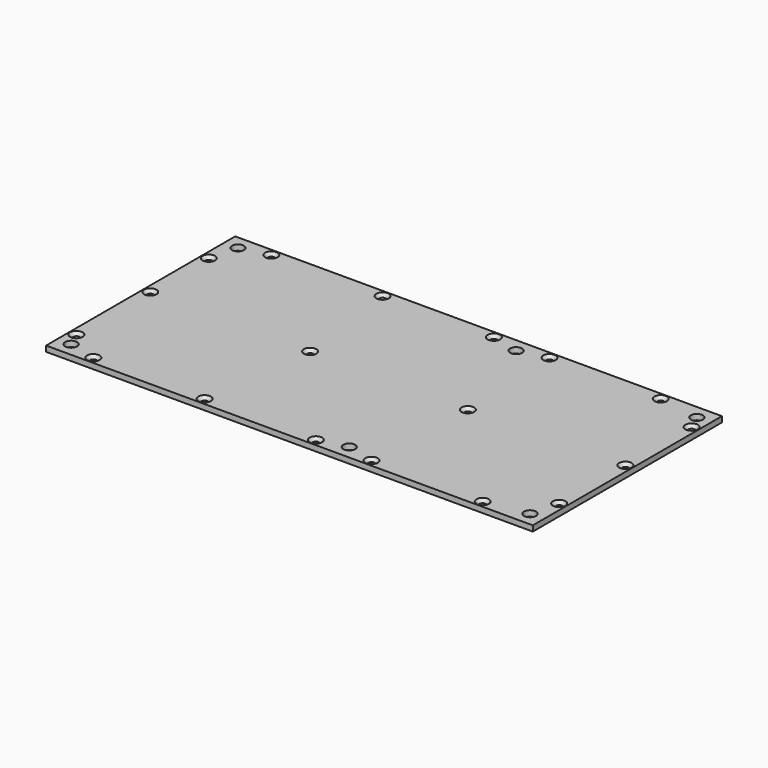
from build123d import *

# Parameters (mm, degrees)
F0_W                 = 175
F0_H                 = 85
F0_R                 = 2.25
F0_R_2               = 1.15
F1_DEPTH             = 2
F2_D                 = 4.3
F4_D                 = 2.3
F4_CSINK_D           = 4.5
F4_CSINK_ANGLE       = 90
F4_ON_F3_D           = 2.3
F4_ON_F3_CSINK_D     = 4.5
F4_ON_F3_CSINK_ANGLE = 90


# Not quite as in the source:
# - ends of sketch curves that miss each other by under 0.0002 mm in the source are joined


with BuildPart() as f1:
    # F0 (on Top) → F1 (new body)
    with BuildSketch(Plane.XY):
        Rectangle(F0_W, F0_H)
        with BuildLine():
            ThreePointArc((-80.499999, -37.5), (-82.499999, -39.5), (-84.499999, -37.5))
            ThreePointArc((-84.499999, -37.5), (-82.4999995, -35.499999), (-80.499999, -37.5))
        make_face(mode=Mode.SUBTRACT)
        with Locations((-72.5, -40)):
            Circle(F0_R, mode=Mode.SUBTRACT)
        with Locations((-85, -32)):
            Circle(F0_R, mode=Mode.SUBTRACT)
        with Locations((-32.5, -40)):
            Circle(F0_R, mode=Mode.SUBTRACT)
        with Locations((7.5, -40)):
            Circle(F0_R, mode=Mode.SUBTRACT)
        with BuildLine():
            ThreePointArc((19.500001, -37.5), (17.500001, -39.5), (15.500001, -37.5))
            ThreePointArc((15.500001, -37.5), (17.5000005, -35.499999), (19.500001, -37.5))
        make_face(mode=Mode.SUBTRACT)
        with Locations((27.5, -40)):
            Circle(F0_R, mode=Mode.SUBTRACT)
        with Locations((67.5, -40)):
            Circle(F0_R, mode=Mode.SUBTRACT)
        with BuildLine():
            ThreePointArc((84.500001, -37.5), (82.500001, -39.5), (80.500001, -37.5))
            ThreePointArc((80.500001, -37.5), (82.5000005, -35.499999), (84.500001, -37.5))
        make_face(mode=Mode.SUBTRACT)
        with Locations((85, -27.5)):
            Circle(F0_R, mode=Mode.SUBTRACT)
        with Locations((-85, 0)):
            Circle(F0_R, mode=Mode.SUBTRACT)
        with Locations((-85, 27.5)):
            Circle(F0_R, mode=Mode.SUBTRACT)
        with BuildLine():
            ThreePointArc((-80.499999, 37.5), (-82.499999, 35.5), (-84.499999, 37.5))
            ThreePointArc((-84.499999, 37.5), (-82.4999995, 39.500001), (-80.499999, 37.5))
        make_face(mode=Mode.SUBTRACT)
        with Locations((-72.5, 40)):
            Circle(F0_R, mode=Mode.SUBTRACT)
        with Locations((-32.5, 40)):
            Circle(F0_R, mode=Mode.SUBTRACT)
        with Locations((85, 0)):
            Circle(F0_R, mode=Mode.SUBTRACT)
        with Locations((7.5, 40)):
            Circle(F0_R, mode=Mode.SUBTRACT)
        with BuildLine():
            ThreePointArc((19.500001, 37.5), (17.500001, 35.5), (15.500001, 37.5))
            ThreePointArc((15.500001, 37.5), (17.5000005, 39.500001), (19.500001, 37.5))
        make_face(mode=Mode.SUBTRACT)
        with Locations((27.5, 40)):
            Circle(F0_R, mode=Mode.SUBTRACT)
        with Locations((85, 24.3)):
            Circle(F0_R, mode=Mode.SUBTRACT)
        with Locations((67.5, 40)):
            Circle(F0_R, mode=Mode.SUBTRACT)
        with BuildLine():
            ThreePointArc((84.500001, 37.5), (82.500001, 35.5), (80.500001, 37.5))
            ThreePointArc((80.500001, 37.5), (82.5000005, 39.500001), (84.500001, 37.5))
        make_face(mode=Mode.SUBTRACT)
        with Locations((-85, 27.5)):
            Circle(F0_R)
        with Locations((-85, 27.5)):
            Circle(F0_R_2, mode=Mode.SUBTRACT)
        with Locations((7.5, 40)):
            Circle(F0_R)
        with Locations((7.5, 40)):
            Circle(F0_R_2, mode=Mode.SUBTRACT)
        with Locations((-32.5, -40)):
            Circle(F0_R)
        with Locations((-32.5, -40)):
            Circle(F0_R_2, mode=Mode.SUBTRACT)
        with Locations((7.5, -40)):
            Circle(F0_R)
        with Locations((7.5, -40)):
            Circle(F0_R_2, mode=Mode.SUBTRACT)
        with Locations((-85, 0)):
            Circle(F0_R)
        with Locations((-85, 0)):
            Circle(F0_R_2, mode=Mode.SUBTRACT)
        with Locations((-32.5, 40)):
            Circle(F0_R)
        with Locations((-32.5, 40)):
            Circle(F0_R_2, mode=Mode.SUBTRACT)
        with Locations((85, 0)):
            Circle(F0_R)
        with Locations((85, 0)):
            Circle(F0_R_2, mode=Mode.SUBTRACT)
        with Locations((-72.5, 40)):
            Circle(F0_R)
        with Locations((-72.5, 40)):
            Circle(F0_R_2, mode=Mode.SUBTRACT)
        with Locations((-85, -32)):
            Circle(F0_R)
        with Locations((-85, -32)):
            Circle(F0_R_2, mode=Mode.SUBTRACT)
        with Locations((-72.5, -40)):
            Circle(F0_R)
        with Locations((-72.5, -40)):
            Circle(F0_R_2, mode=Mode.SUBTRACT)
        with Locations((27.5, 40)):
            Circle(F0_R)
        with Locations((27.5, 40)):
            Circle(F0_R_2, mode=Mode.SUBTRACT)
        with Locations((27.5, -40)):
            Circle(F0_R)
        with Locations((27.5, -40)):
            Circle(F0_R_2, mode=Mode.SUBTRACT)
        with Locations((67.5, 40)):
            Circle(F0_R)
        with Locations((67.5, 40)):
            Circle(F0_R_2, mode=Mode.SUBTRACT)
        with Locations((85, 24.3)):
            Circle(F0_R)
        with Locations((85, 24.3)):
            Circle(F0_R_2, mode=Mode.SUBTRACT)
        with Locations((67.5, -40)):
            Circle(F0_R)
        with Locations((67.5, -40)):
            Circle(F0_R_2, mode=Mode.SUBTRACT)
        with Locations((85, -27.5)):
            Circle(F0_R)
        with Locations((85, -27.5)):
            Circle(F0_R_2, mode=Mode.SUBTRACT)
        with BuildLine():
            ThreePointArc((-80.499999, -37.499999), (-82.4999995, -35.499999), (-84.499999, -37.5))
            ThreePointArc((-84.499999, -37.5), (-82.499999, -39.5), (-80.499999, -37.499999))
        make_face()
        with BuildLine():
            ThreePointArc((19.500001, -37.499999), (17.5000005, -35.499999), (15.500001, -37.5))
            ThreePointArc((15.500001, -37.5), (17.500001, -39.5), (19.500001, -37.499999))
        make_face()
        with BuildLine():
            ThreePointArc((84.500001, 37.500001), (82.5000005, 39.500001), (80.500001, 37.5))
            ThreePointArc((80.500001, 37.5), (82.500001, 35.5), (84.500001, 37.500001))
        make_face()
        with BuildLine():
            ThreePointArc((19.500001, 37.500001), (17.5000005, 39.500001), (15.500001, 37.5))
            ThreePointArc((15.500001, 37.5), (17.500001, 35.5), (19.500001, 37.500001))
        make_face()
        with BuildLine():
            ThreePointArc((-80.499999, 37.500001), (-82.4999995, 39.500001), (-84.499999, 37.5))
            ThreePointArc((-84.499999, 37.5), (-82.499999, 35.5), (-80.499999, 37.500001))
        make_face()
        with BuildLine():
            ThreePointArc((84.500001, -37.499999), (82.5000005, -35.499999), (80.500001, -37.5))
            ThreePointArc((80.500001, -37.5), (82.500001, -39.5), (84.500001, -37.499999))
        make_face()
        with Locations((-85, 27.5)):
            Circle(F0_R_2)
        with Locations((85, 24.3)):
            Circle(F0_R_2)
        with Locations((-85, -32)):
            Circle(F0_R_2)
        with Locations((-72.5, -40)):
            Circle(F0_R_2)
        with Locations((-32.5, -40)):
            Circle(F0_R_2)
        with Locations((7.5, -40)):
            Circle(F0_R_2)
        with Locations((-72.5, 40)):
            Circle(F0_R_2)
        with Locations((7.5, 40)):
            Circle(F0_R_2)
        with Locations((-32.5, 40)):
            Circle(F0_R_2)
        with Locations((85, 0)):
            Circle(F0_R_2)
        with Locations((27.5, -40)):
            Circle(F0_R_2)
        with Locations((-85, 0)):
            Circle(F0_R_2)
        with Locations((67.5, 40)):
            Circle(F0_R_2)
        with Locations((27.5, 40)):
            Circle(F0_R_2)
        with Locations((67.5, -40)):
            Circle(F0_R_2)
        with Locations((85, -27.5)):
            Circle(F0_R_2)
    extrude(amount=-F1_DEPTH)

    # F2 (through all)
    with Locations(Plane.XY):
        with Locations((-82.499999, 37.5), (17.500001, 37.5), (82.500001, 37.5), (82.500001, -37.5), (-82.499999, -37.5), (17.500001, -37.5)):
            Hole(F2_D / 2)

    # F4 (through all)
    with Locations(Plane.XY):
        with Locations((-85, -32), (-72.5, -40), (-85, 27.5), (-72.5, 40), (-32.5, -40), (7.5, -40), (27.5, -40), (67.5, -40), (-32.5, 40), (7.5, 40), (27.5, 40), (67.5, 40), (85, -27.5)):
            CounterSinkHole(F4_D / 2, F4_CSINK_D / 2, counter_sink_angle=F4_CSINK_ANGLE)

    # F4 on F3 (through all)
    with Locations(Plane.XY):
        with Locations((85, 32), (85, 2.25), (-85, 1.2), (-27.35, 1), (29.35, 1)):
            CounterSinkHole(F4_ON_F3_D / 2, F4_ON_F3_CSINK_D / 2, counter_sink_angle=F4_ON_F3_CSINK_ANGLE)


solid = f1.part
